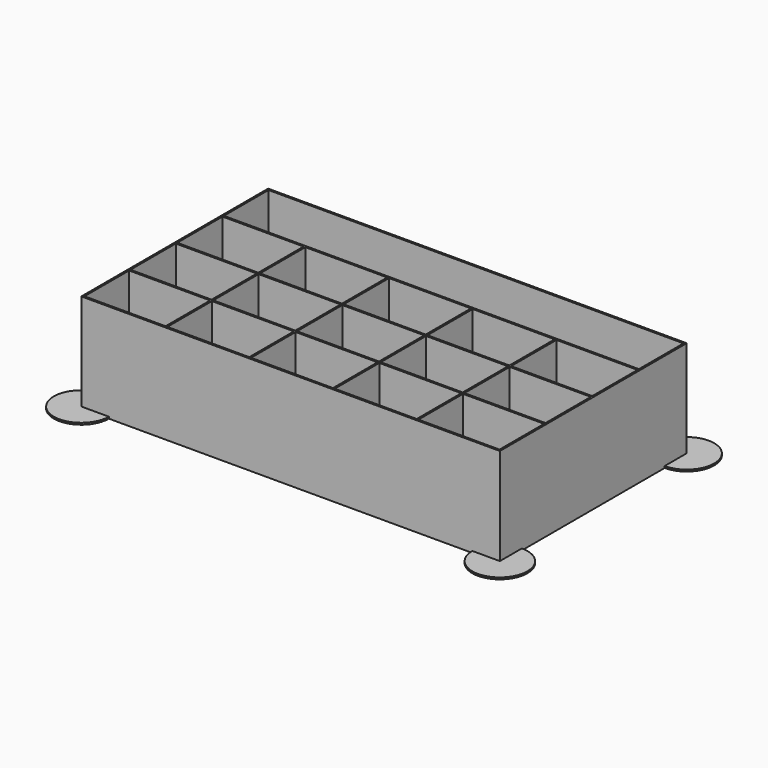
from build123d import *

# Parameters (mm, degrees)
F0_W     = 190
F0_H     = 106
F1_DEPTH = 0.8
F2_W     = 190
F2_H     = 106
F2_W_2   = 36.8
F2_H_2   = 25.3
F2_W_3   = 37.2
F2_H_3   = 25.7
F2_W_4   = 188.4
F3_DEPTH = 44
F4_R     = 12.5
F5_DEPTH = 0.8


# Not quite as in the source:
# - a feature names something its author has since deleted; it is built from what else it names


with BuildPart() as f1:
    # F0 (on Top) → F1 (new body)
    with BuildSketch(Plane.XY):
        with Locations((-95, 53)):
            Rectangle(F0_W, F0_H)
    extrude(amount=F1_DEPTH)

    # F2 (on face) → F3 (join)
    with BuildSketch(Plane.XY.offset(0.8)):
        with Locations((-95, 53)):
            Rectangle(F2_W, F2_H)
        with Locations((-170.8, 13.45)):
            Rectangle(F2_W_2, F2_H_2, mode=Mode.SUBTRACT)
        with Locations((-133, 13.45)):
            Rectangle(F2_W_3, F2_H_2, mode=Mode.SUBTRACT)
        with Locations((-170.8, 39.75)):
            Rectangle(F2_W_2, F2_H_3, mode=Mode.SUBTRACT)
        with Locations((-133, 39.75)):
            Rectangle(F2_W_3, F2_H_3, mode=Mode.SUBTRACT)
        with Locations((-95, 13.45)):
            Rectangle(F2_W_3, F2_H_2, mode=Mode.SUBTRACT)
        with Locations((-57, 13.45)):
            Rectangle(F2_W_3, F2_H_2, mode=Mode.SUBTRACT)
        with Locations((-19.2, 13.45)):
            Rectangle(F2_W_2, F2_H_2, mode=Mode.SUBTRACT)
        with Locations((-95, 39.75)):
            Rectangle(F2_W_3, F2_H_3, mode=Mode.SUBTRACT)
        with Locations((-57, 39.75)):
            Rectangle(F2_W_3, F2_H_3, mode=Mode.SUBTRACT)
        with Locations((-19.2, 39.75)):
            Rectangle(F2_W_2, F2_H_3, mode=Mode.SUBTRACT)
        with Locations((-170.8, 66.25)):
            Rectangle(F2_W_2, F2_H_3, mode=Mode.SUBTRACT)
        with Locations((-133, 66.25)):
            Rectangle(F2_W_3, F2_H_3, mode=Mode.SUBTRACT)
        with Locations((-95, 66.25)):
            Rectangle(F2_W_3, F2_H_3, mode=Mode.SUBTRACT)
        with Locations((-57, 66.25)):
            Rectangle(F2_W_3, F2_H_3, mode=Mode.SUBTRACT)
        with Locations((-19.2, 66.25)):
            Rectangle(F2_W_2, F2_H_3, mode=Mode.SUBTRACT)
        with Locations((-95, 92.55)):
            Rectangle(F2_W_4, F2_H_2, mode=Mode.SUBTRACT)
    extrude(amount=F3_DEPTH)

    # F4 (on face) → F5 (join)
    with BuildSketch(Plane(origin=(0, 0, 0), x_dir=(1, 0, 0), z_dir=(0, 0, -1))):
        Circle(F4_R)
        with Locations((-190, 0)):
            Circle(F4_R)
        with Locations((-190, -106)):
            Circle(F4_R)
        with Locations((0, -106)):
            Circle(F4_R)
    extrude(amount=-F5_DEPTH)


solid = f1.part
